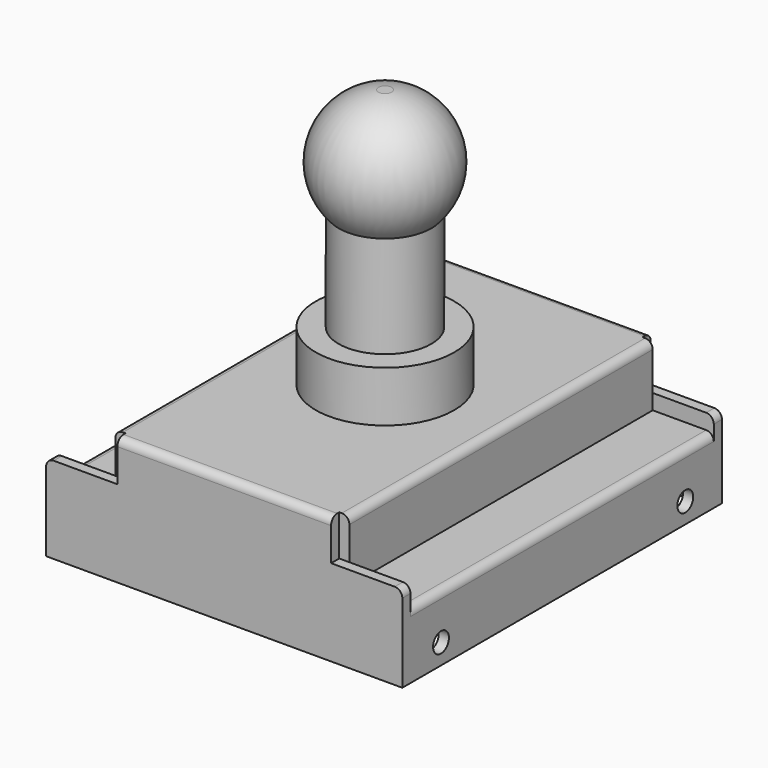
from build123d import *

# Parameters (mm, degrees)
F1_W      = 70
F1_H      = 25
F2_DEPTH  = 78.5
F3_W      = 15
F3_H      = 10
F4_DEPTH  = 2
F5_W      = 15
F5_H      = 10
F6_DEPTH  = 2
F7_W      = 17.4621326589
F7_H      = 19.2356310288
F8_DEPTH  = 74.5
F10_T     = -2
F11_R     = 1.5
F12_R     = 1.95
F13_DEPTH = 70.001
F14_R     = 13.6
F15_DEPTH = 10
F16_R     = 9.1
F17_DEPTH = 20
F18_R     = 12.5
F19_DEPTH = 21


# Not quite as in the source:
# - a feature of the source that left no trace in its solid (it failed there, or was rolled back) is left out


with BuildPart() as f2:
    # F1 (on offset) → F2 (new body)
    with BuildSketch(Plane.XZ.offset(39.5)):
        with Locations((0, 12.5)):
            Rectangle(F1_W, F1_H)
    extrude(amount=-F2_DEPTH)

    # F3 (on face) → F4 (cut)
    with BuildSketch(Plane.XZ.offset(39.5)):
        with Locations((-28.5, 22)):
            Rectangle(F3_W, F3_H)
        with Locations((28.5, 22)):
            Rectangle(F3_W, F3_H)
    extrude(amount=-F4_DEPTH, mode=Mode.SUBTRACT)

    # F5 (on face) → F6 (cut)
    with BuildSketch(Plane(origin=(0, 39, 0), x_dir=(-1, 0, 0), z_dir=(0, 1, 0))):
        with Locations((-28.5, 21)):
            Rectangle(F5_W, F5_H)
        with Locations((28.5, 21)):
            Rectangle(F5_W, F5_H)
    extrude(amount=-F6_DEPTH, mode=Mode.SUBTRACT)

    # F7 (on face) → F8 (cut)
    with BuildSketch(Plane.XZ.offset(37.5)):
        with Locations((-31.7310663294, 22.6178155144)):
            Rectangle(F7_W, F7_H)
        with Locations((31.7310663294, 22.6178155144)):
            Rectangle(F7_W, F7_H)
    extrude(amount=-F8_DEPTH, mode=Mode.SUBTRACT)

    # F10: a shell. OpenCascade refuses it in one call, so the cavity is built on its own and cut out:
    # the body offset inwards by the wall thickness, plus a prism from it out through each open face.
    f10_core = offset(f2.part, amount=F10_T, kind=Kind.INTERSECTION, mode=Mode.PRIVATE)
    f10_exits = [f10_core.faces().sort_by_distance(p)[0] for p in [
        (0, -0.25, 2),
    ]]
    add(f10_core, mode=Mode.SUBTRACT)
    extrude(f10_exits, amount=-F10_T, mode=Mode.SUBTRACT)

    # F11
    f11_edges = [f2.edges().sort_by_distance(p)[0] for p in [
        (21, -0.25, 11),
        (-21, -0.25, 11),
        (-35, -38.5, 17),
        (-35, 38, 16),
        (-35, -0.25, 13),
        (-23, -0.25, 25),
        (0, -39.5, 25),
        (0, 39, 25),
        (23, -0.25, 25),
        (35, -38.5, 17),
        (35, -0.25, 13),
        (35, 38, 16),
    ]]
    fillet(f11_edges, radius=F11_R)

    # F12 (on face) → F13 (cut, through all)
    with BuildSketch(Plane.YZ.offset(35)):
        with Locations((-30, 4)):
            Circle(F12_R)
        with Locations((30, 4)):
            Circle(F12_R)
    extrude(amount=-F13_DEPTH, mode=Mode.SUBTRACT)

    # F14 (on face) → F15 (join)
    with BuildSketch(Plane.XY.offset(25)):
        Circle(F14_R)
    extrude(amount=F15_DEPTH)

    # F16 (on face) → F17 (join)
    with BuildSketch(Plane.XY.offset(35)):
        Circle(F16_R)
    extrude(amount=F17_DEPTH)

    # F18 (on face) → F19 (join)
    with BuildSketch(Plane.XY.offset(55)):
        Circle(F18_R)
    extrude(amount=F19_DEPTH)

    # F20 (on Front) → F21 (revolve, cut)
    with BuildSketch(Plane.XZ):
        with BuildLine():
            ThreePointArc((0, 76.0678347956), (11.4737550942, 68.5243920963), (9.100375697, 54.9996867776))
            Line((9.100375697, 54.9996867776), (14.105156064, 54.9996867776))
            Line((14.105156064, 54.9996867776), (14.105156064, 76.9773796201))
            Line((14.105156064, 76.9773796201), (0, 76.9773796201))
            Line((0, 76.9773796201), (0, 76.0678347956))
        make_face()
    revolve(axis=Axis((0, 0, 76.5226072078), (0, 0, -1)), mode=Mode.SUBTRACT)


solid = f2.part
